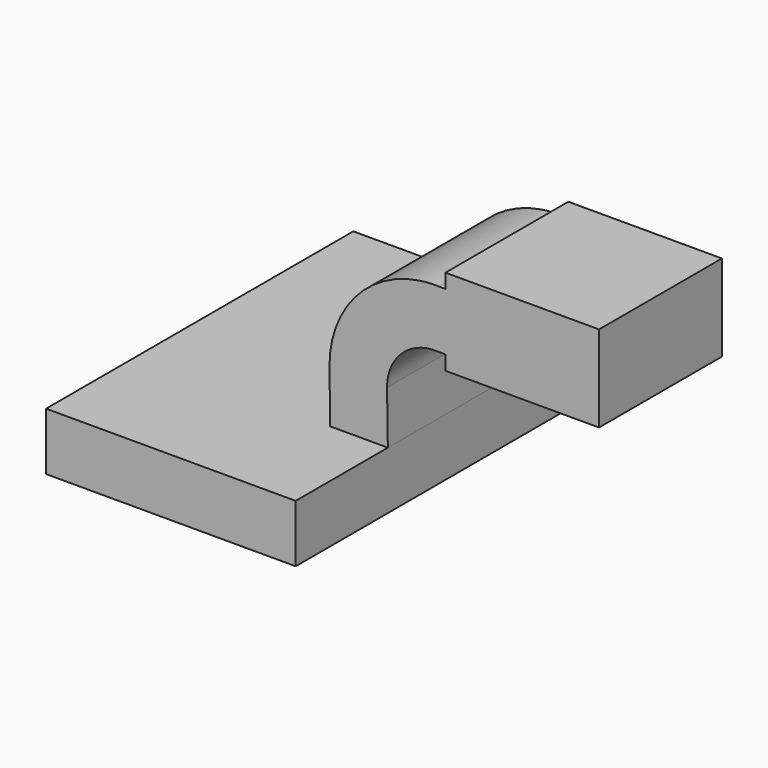
from build123d import *

# Parameters (mm, degrees)
F1_DEPTH = 63.5
F0_W     = 25.4
F0_H     = 19.05
F0_H_2   = 4.7752
F0_H_3   = 4.7498
F2_DEPTH = 25.4


# Not quite as in the source:
# - a feature of the source that left no trace in its solid (it failed there, or was rolled back) is left out


with BuildPart() as f1:
    # F0 (on Front) → F1 (new body, symmetric)
    with BuildSketch(Plane.XZ):
        Polygon((41.275, -9.525), (41.275, 9.525), (22.2228064707, 9.525), (-41.275, 9.525), (-41.275, -9.525), align=None)
    extrude(amount=F1_DEPTH, both=True)

    # F0 (on Front) → F2 (join, symmetric)
    with BuildSketch(Plane.XZ):
        with BuildLine():
            add(Edge.make_bspline(
                [(51.4118423464, 61.5169892273), (53.7469843796, 61.749049716), (56.003883812, 61.8875588148), (58.1631200711, 61.9252)],
                knots=[105.6886926289, 105.6886926289, 105.6886926289, 105.6886926289, 112.3998251036, 112.3998251036, 112.3998251036, 112.3998251036], degree=3))
            ThreePointArc((58.1631200711, 61.9252), (54.7775761271, 61.8849118409), (51.4118423464, 61.5169892273))
        make_face()
        Polygon((41.275, -9.525), (41.275, 9.525), (22.2228064707, 9.525), (-41.275, 9.525), (-41.275, -9.525), align=None)
        with BuildLine():
            Line((41.275, 9.525), (41.0106324272, 26.945333009))
            ThreePointArc((41.0106324272, 26.945333009), (45.9404876374, 38.5224332318), (57.7466785314, 42.8752))
            Line((57.7466785314, 42.8752), (60.325, 42.8752))
            Line((60.325, 42.8752), (60.325, 61.9252))
            Line((60.325, 61.9252), (58.1631200711, 61.9252))
            add(Edge.make_bspline(
                [(51.4118423464, 61.5169892273), (53.7469843796, 61.749049716), (56.003883812, 61.8875588148), (58.1631200711, 61.9252)],
                knots=[105.6886926289, 105.6886926289, 105.6886926289, 105.6886926289, 112.3998251036, 112.3998251036, 112.3998251036, 112.3998251036], degree=3))
            ThreePointArc((51.4118423464, 61.5169892273), (30.2314207387, 49.5916736898), (21.9616330248, 26.7348580473))
            Line((21.9616330248, 26.7348580473), (22.2228064707, 9.525))
            Line((22.2228064707, 9.525), (41.275, 9.525))
        make_face()
        with Locations((73.025, 52.4002)):
            Rectangle(F0_W, F0_H)
        with Locations((73.025, 40.4876)):
            Rectangle(F0_W, F0_H_2)
        Polygon((85.725, 61.9252), (85.725, 42.8752), (85.725, 38.1), (111.125, 38.1), (111.125, 66.675), (85.725, 66.675), align=None)
        with Locations((73.025, 64.3001)):
            Rectangle(F0_W, F0_H_3)
    extrude(amount=F2_DEPTH, both=True)


solid = f1.part
